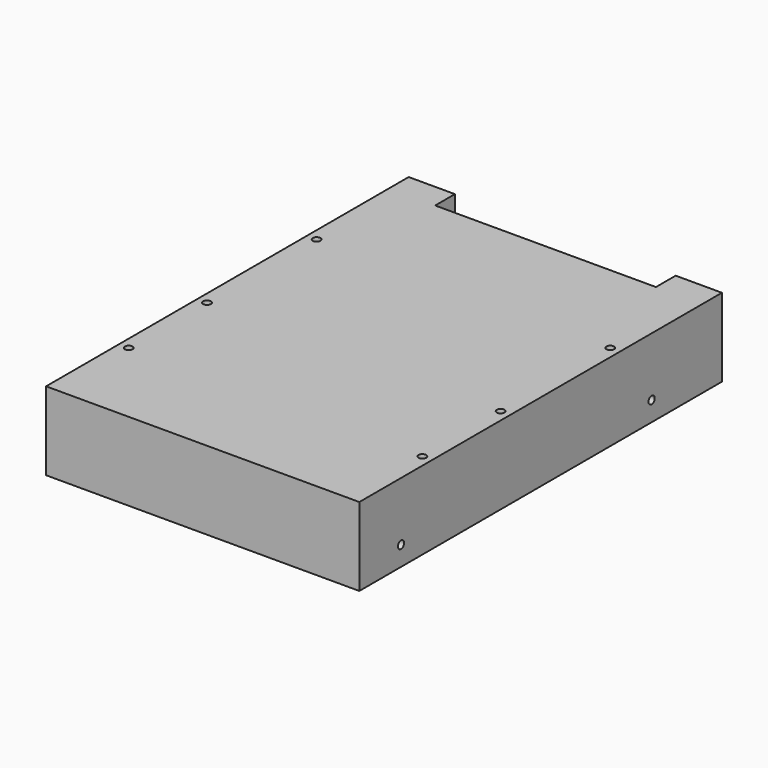
from build123d import *

# Parameters (mm, degrees)
F0_W     = 101.6
F0_H     = 147
F1_DEPTH = 25.4
F2_R     = 1.25
F2_W     = 71.6
F2_H     = 8
F3_DEPTH = 10
F4_R     = 1.25
F5_DEPTH = 10


# Not quite as in the source:
# - a pattern or mirror of a feature is missing from the dataset's text; its kind, count and spacing are read off the source's solid


with BuildPart() as f1:
    # F0 (on Top) → F1 (new body)
    with BuildSketch(Plane.XY):
        with Locations((50.8, 73.5)):
            Rectangle(F0_W, F0_H)
    extrude(amount=F1_DEPTH)

    # F2 (on face) → F3 (cut)
    with BuildSketch(Plane.XY.offset(25.4)):
        with Locations((3.18, 29.52)):
            Circle(F2_R)
        with Locations((3.18, 61.27)):
            Circle(F2_R)
        with Locations((3.18, 105.72)):
            Circle(F2_R)
        with Locations((98.42, 29.52)):
            Circle(F2_R)
        with Locations((98.42, 61.27)):
            Circle(F2_R)
        with Locations((98.42, 105.72)):
            Circle(F2_R)
        with Locations((50.8, 143)):
            Rectangle(F2_W, F2_H)
    extrude(amount=-F3_DEPTH, mode=Mode.SUBTRACT)

    # F4 (on face) → F5 (cut)
    with BuildSketch(Plane(origin=(0, 0, 0), x_dir=(0, -1, 0), z_dir=(-1, 0, 0))):
        with Locations((-118.5, 6.35)):
            Circle(F4_R)
        with Locations((-16.9, 6.35)):
            Circle(F4_R)
    f5 = extrude(amount=-F5_DEPTH, mode=Mode.SUBTRACT)

    # F5_copies: F5 across plane
    add(f5.mirror(Plane(origin=(50.8, 0, 0), x_dir=(0, 0, 1), z_dir=(1, 0, 0))), mode=Mode.SUBTRACT)


solid = f1.part
